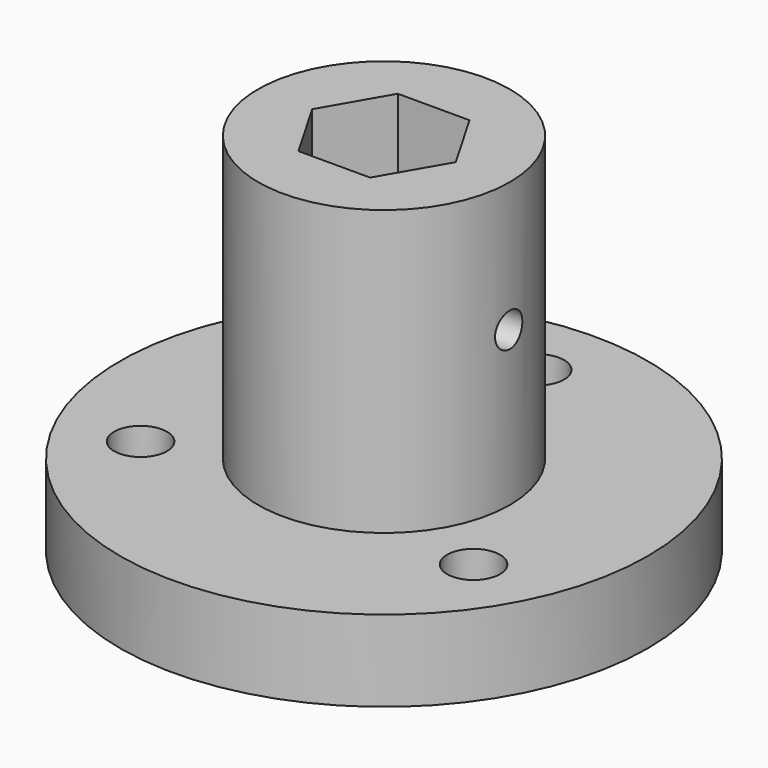
from build123d import *

# Parameters (mm, degrees)
F0_R      = 32.5
F1_DEPTH  = 10
F2_R      = 15.5
F3_DEPTH  = 35
F5_R      = 4.8
F6_DEPTH  = 45.001
F7_R      = 4.8
F8_DEPTH  = 34
F10_DEPTH = 22
F12_DEPTH = 6
F13_R     = 2.1
F14_DEPTH = 25
F15_R     = 3.25
F16_DEPTH = 45.0010001
F17_R     = 3.25
F18_DEPTH = 2.5


# Not quite as in the source:
# - a feature names something its author has since deleted; it is built from what else it names


with BuildPart() as f1:
    # F0 (on Top) → F1 (new body)
    with BuildSketch(Plane.XY):
        Circle(F0_R)
    extrude(amount=F1_DEPTH)

    # F2 (on face) → F3 (join)
    with BuildSketch(Plane.XY.offset(10)):
        Circle(F2_R)
    extrude(amount=F3_DEPTH)

    # F5 (on face) → F6 (cut, through all)
    with BuildSketch(Plane.XY):
        Circle(F5_R)
    extrude(amount=F6_DEPTH, mode=Mode.SUBTRACT)

    # F7 (on face) → F8 (cut)
    with BuildSketch(Plane.XY.offset(45)):
        Polygon((3.3412309145, -6.2007668324), (7.040637057, -0.2067925644), (3.6994061426, 5.993974268), (-3.3412309145, 6.2007668324), (-7.040637057, 0.2067925644), (-3.6994061426, -5.993974268), align=None)
        Circle(F7_R, mode=Mode.SUBTRACT)
    extrude(amount=-F8_DEPTH, mode=Mode.SUBTRACT)

    # F9 (on face) → F10 (cut)
    with BuildSketch(Plane.XY.offset(45)):
        Polygon((-4.4167295593, -7.65), (4.4167295593, -7.65), (8.8334591186, 0), (4.4167295593, 7.65), (-4.4167295593, 7.65), (-8.8334591186, 0), align=None)
        Polygon((3.3412309145, -6.2007668324), (-3.6994061426, -5.993974268), (-7.040637057, 0.2067925644), (-3.3412309145, 6.2007668324), (3.6994061426, 5.993974268), (7.040637057, -0.2067925644), align=None, mode=Mode.SUBTRACT)
    extrude(amount=-F10_DEPTH, mode=Mode.SUBTRACT)

    # F11 (on face) → F12 (cut)
    with BuildSketch(Plane.XY):
        Polygon((-15.35, -8.8623266321), (-20.5, -5.8889727457), (-25.65, -8.8623266321), (-25.65, -14.8090344047), (-20.5, -17.782388291), (-15.35, -14.8090344047), align=None)
        Polygon((0, 29.6180688094), (-5.15, 26.6447149231), (-5.15, 20.6980071504), (0, 17.7246532641), (5.15, 20.6980071504), (5.15, 26.6447149231), align=None)
        Polygon((25.65, -14.8090344047), (25.65, -8.8623266321), (20.5, -5.8889727457), (15.35, -8.8623266321), (15.35, -14.8090344047), (20.5, -17.782388291), align=None)
    extrude(amount=F12_DEPTH, mode=Mode.SUBTRACT)

    # F13 (on Right) → F14 (cut, symmetric)
    with BuildSketch(Plane.YZ):
        with Locations((0, 29)):
            Circle(F13_R)
    extrude(amount=F14_DEPTH, both=True, mode=Mode.SUBTRACT)

    # F15 (on face) → F16 (cut, through all)
    with BuildSketch(Plane.XY):
        with Locations((-20.5, -11.8356805184)):
            Circle(F15_R)
        with Locations((0, 23.6713610368)):
            Circle(F15_R)
        with Locations((20.5, -11.8356805184)):
            Circle(F15_R)
    extrude(amount=F16_DEPTH, mode=Mode.SUBTRACT)

    # F17 (on face) → F18 (cut)
    with BuildSketch(Plane.XY):
        with BuildLine():
            ThreePointArc((-25.1062968267, -16.4217495916), (-18.0191664076, -17.8436306419), (-14, -11.8356805184))
            ThreePointArc((-14, -11.8356805184), (-21.3555101482, -5.3922262905), (-26.7748007343, -13.5318160511))
            ThreePointArc((-26.7748007343, -13.5318160511), (-25.9807621135, -15), (-25.1062968267, -16.4217495916))
        make_face()
        with Locations((-20.5, -11.8356805184)):
            Circle(F17_R, mode=Mode.SUBTRACT)
        with BuildLine():
            ThreePointArc((-25.1062968267, -16.4217495916), (-25.9807621135, -15), (-26.7748007343, -13.5318160511))
            ThreePointArc((-26.7748007343, -13.5318160511), (-26.1291651246, -15.0856805184), (-25.1062968267, -16.4217495916))
        make_face()
        with BuildLine():
            ThreePointArc((1.6685039075, 29.9535656427), (0, 30), (-1.6685039075, 29.9535656427))
            ThreePointArc((-1.6685039075, 29.9535656427), (-3.9626206354, 18.5189210614), (6.5, 23.6713610368))
            ThreePointArc((6.5, 23.6713610368), (5.1524399753, 27.6339816722), (1.6685039075, 29.9535656427))
        make_face()
        with BuildLine():
            ThreePointArc((1.6685039075, 29.9535656427), (0, 30.1713610368), (-1.6685039075, 29.9535656427))
            ThreePointArc((-1.6685039075, 29.9535656427), (0, 30), (1.6685039075, 29.9535656427))
        make_face()
        with BuildLine():
            ThreePointArc((26.7748007343, -13.5318160511), (25.9807621135, -15), (25.1062968267, -16.4217495916))
            ThreePointArc((25.1062968267, -16.4217495916), (26.1291651246, -15.0856805184), (26.7748007343, -13.5318160511))
        make_face()
        with BuildLine():
            ThreePointArc((27, -11.8356805184), (14.4920498765, -9.354846926), (25.1062968267, -16.4217495916))
            ThreePointArc((25.1062968267, -16.4217495916), (25.9807621135, -15), (26.7748007343, -13.5318160511))
            ThreePointArc((26.7748007343, -13.5318160511), (26.9434542278, -12.6911906666), (27, -11.8356805184))
        make_face()
    extrude(amount=F18_DEPTH, mode=Mode.SUBTRACT)


solid = f1.part
